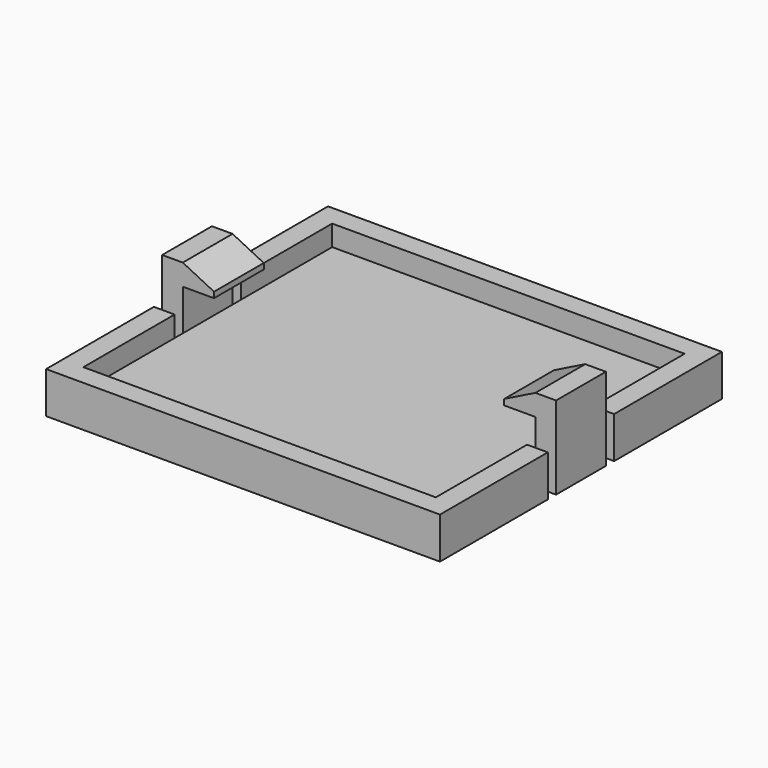
from build123d import *

# Parameters (mm, degrees)
F1_DEPTH  = 1
F2_DEPTH  = 2
F0_W      = 1
F0_H      = 3
F3_DEPTH  = 4
F4_W      = 3
F4_H      = 1.0236278605
F5_DEPTH  = 1.5
F7_DEPTH  = 3
F9_DEPTH  = 2
F10_W     = 8.5
F10_H     = 15
F11_DEPTH = 2


# Not quite as in the source:
# - a feature names something its author has since deleted; it is built from what else it names


with BuildPart() as f1:
    # F0 (on Top) → F1 (new body)
    with BuildSketch(Plane.XY):
        Polygon((-8.5, 7.5), (-8.5, 2), (-8.5, 1.5), (-8.5, -1.5), (-8.5, -2), (-8.5, -7.5), (8.5, -7.5), (8.5, 7.5), align=None)
    extrude(amount=F1_DEPTH)

    # F0 (on Top) → F2 (join)
    with BuildSketch(Plane.XY):
        Polygon((9.5, 8.5), (-9.5, 8.5), (-9.5, 2), (-8.5, 2), (-8.5, 7.5), (8.5, 7.5), (8.5, -7.5), (-8.5, -7.5), (-8.5, -2), (-9.5, -2), (-9.5, -8.5), (9.5, -8.5), align=None)
    extrude(amount=F2_DEPTH)

    # F0 (on Top) → F3 (join)
    with BuildSketch(Plane.XY):
        with Locations((-9, 0)):
            Rectangle(F0_W, F0_H)
    extrude(amount=F3_DEPTH)

    # F4 (on face) → F5 (join)
    with BuildSketch(Plane.YZ.offset(-8.5)):
        with Locations((0, 3.4881860698)):
            Rectangle(F4_W, F4_H)
    extrude(amount=F5_DEPTH)

    # F6 (on face) → F7 (cut)
    with BuildSketch(Plane.XZ.offset(1.5)):
        Polygon((-8.5056265816, 4), (-7, 3.2529253513), (-7, 4), align=None)
    extrude(amount=-F7_DEPTH, mode=Mode.SUBTRACT)

    # F8 (on face) → F9 (cut)
    with BuildSketch(Plane.XY.offset(2)):
        Polygon((9.5, 8.5), (0, 8.5), (0, 7.5), (8.5, 7.5), (8.5, -7.5), (0, -7.5), (0, -8.5), (9.5, -8.5), align=None)
    extrude(amount=-F9_DEPTH, mode=Mode.SUBTRACT)

    # F10 (on face) → F11 (cut)
    with BuildSketch(Plane.XY.offset(1)):
        with Locations((4.25, 0)):
            Rectangle(F10_W, F10_H)
    extrude(amount=-F11_DEPTH, mode=Mode.SUBTRACT)

    # F12: F1 across plane


with BuildPart() as f1_1:
    add(f1.part)
    add(f1.part.mirror(Plane.YZ))


solid = f1_1.part
